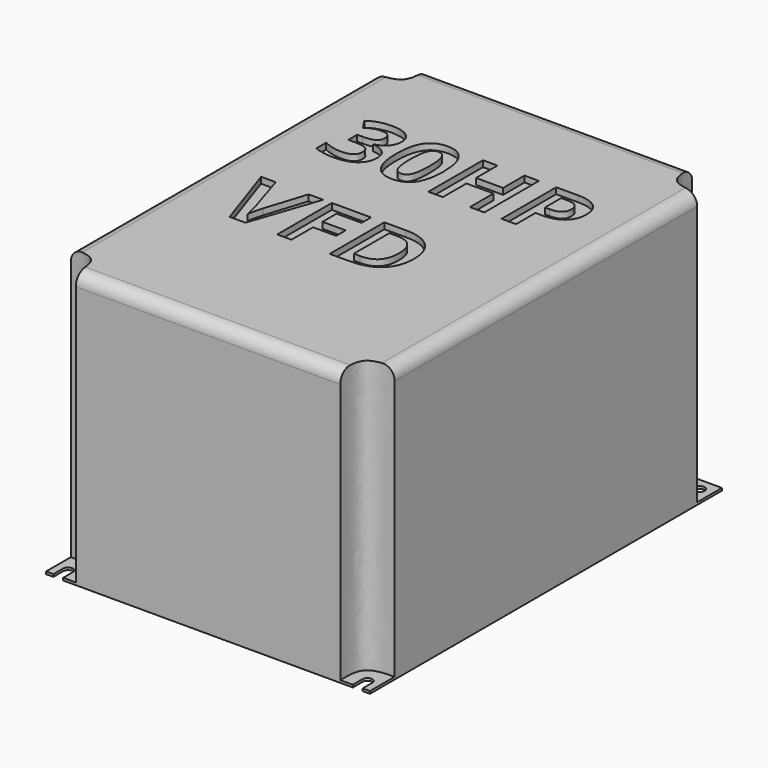
from build123d import *

# Parameters (mm, degrees)
F0_R         = 4
F1_DEPTH     = 2
F2_DEPTH     = 225
F3_R         = 10
F4_TEXT_SIZE = 78.2922502905
F5_DEPTH     = 5


# Not quite as in the source:
# - Text() gives the source's letters only with a copy of the font that has no kerning and outlines rounded to 1/6400 em; it was checked with that copy


with BuildPart() as f1:
    # F0 (on Top) → F1 (new body)
    with BuildSketch(Plane.XY):
        with BuildLine():
            Line((-108.2113981247, 180), (-132.5, 180))
            Line((-132.5, 180), (-132.5, 154.7320783138))
            add(Edge.make_bspline(
                [(-108.2113981247, 180), (-108.2113981247, 171.2072445138), (-108.3167336436, 156.7946357948), (-122.3416605587, 154.7320783138), (-132.5, 154.7320783138)],
                knots=[0, 0, 0, 0, 0.4931140285, 1, 1, 1, 1], degree=3))
        make_face()
        with Locations((-122.5, 170)):
            Circle(F0_R, mode=Mode.SUBTRACT)
        with BuildLine():
            Line((108.2113981247, 180), (-108.2113981247, 180))
            add(Edge.make_bspline(
                [(-108.2113981247, 180), (-108.2113981247, 171.2072445138), (-108.3167336436, 156.7946357948), (-122.3416605587, 154.7320783138), (-132.5, 154.7320783138)],
                knots=[0, 0, 0, 0, 0.4931140285, 1, 1, 1, 1], degree=3))
            Line((-132.5, 154.7320783138), (-132.5, -154.7320783138))
            add(Edge.make_bspline(
                [(-108.2113981247, -180), (-108.2113981247, -171.2072445138), (-108.3167336436, -156.7946357948), (-122.3416605587, -154.7320783138), (-132.5, -154.7320783138)],
                knots=[0, 0, 0, 0, 0.4931140285, 1, 1, 1, 1], degree=3))
            Line((-108.2113981247, -180), (108.2113981247, -180))
            add(Edge.make_bspline(
                [(108.2113981247, -180), (108.2113981247, -171.2072445138), (108.3167336436, -156.7946357948), (122.3416605587, -154.7320783138), (132.5, -154.7320783138)],
                knots=[0, 0, 0, 0, 0.4931140285, 1, 1, 1, 1], degree=3))
            Line((132.5, -154.7320783138), (132.5, 154.7320783138))
            add(Edge.make_bspline(
                [(108.2113981247, 180), (108.2113981247, 171.2072445138), (108.3167336436, 156.7946357948), (122.3416605587, 154.7320783138), (132.5, 154.7320783138)],
                knots=[0, 0, 0, 0, 0.4931140285, 1, 1, 1, 1], degree=3))
        make_face()
        with BuildLine():
            Line((132.5, 180), (108.2113981247, 180))
            add(Edge.make_bspline(
                [(108.2113981247, 180), (108.2113981247, 171.2072445138), (108.3167336436, 156.7946357948), (122.3416605587, 154.7320783138), (132.5, 154.7320783138)],
                knots=[0, 0, 0, 0, 0.4931140285, 1, 1, 1, 1], degree=3))
            Line((132.5, 154.7320783138), (132.5, 180))
        make_face()
        with Locations((122.5, 170)):
            Circle(F0_R, mode=Mode.SUBTRACT)
        with BuildLine():
            Line((132.5, -180), (132.5, -154.7320783138))
            add(Edge.make_bspline(
                [(108.2113981247, -180), (108.2113981247, -171.2072445138), (108.3167336436, -156.7946357948), (122.3416605587, -154.7320783138), (132.5, -154.7320783138)],
                knots=[0, 0, 0, 0, 0.4931140285, 1, 1, 1, 1], degree=3))
            Line((108.2113981247, -180), (118.5, -180))
            Line((118.5, -180), (118.5, -170))
            ThreePointArc((118.5, -170), (122.5, -166), (126.5, -170))
            Line((126.5, -170), (126.5, -180))
            Line((126.5, -180), (132.5, -180))
        make_face()
        with BuildLine():
            add(Edge.make_bspline(
                [(-108.2113981247, -180), (-108.2113981247, -171.2072445138), (-108.3167336436, -156.7946357948), (-122.3416605587, -154.7320783138), (-132.5, -154.7320783138)],
                knots=[0, 0, 0, 0, 0.4931140285, 1, 1, 1, 1], degree=3))
            Line((-132.5, -154.7320783138), (-132.5, -180))
            Line((-132.5, -180), (-126.5, -180))
            Line((-126.5, -180), (-126.5, -170))
            ThreePointArc((-126.5, -170), (-122.5, -166), (-118.5, -170))
            Line((-118.5, -170), (-118.5, -180))
            Line((-118.5, -180), (-108.2113981247, -180))
        make_face()
    extrude(amount=F1_DEPTH)

    # F0 (on Top) → F2 (join)
    with BuildSketch(Plane.XY):
        with BuildLine():
            Line((108.2113981247, 180), (-108.2113981247, 180))
            add(Edge.make_bspline(
                [(-108.2113981247, 180), (-108.2113981247, 171.2072445138), (-108.3167336436, 156.7946357948), (-122.3416605587, 154.7320783138), (-132.5, 154.7320783138)],
                knots=[0, 0, 0, 0, 0.4931140285, 1, 1, 1, 1], degree=3))
            Line((-132.5, 154.7320783138), (-132.5, -154.7320783138))
            add(Edge.make_bspline(
                [(-108.2113981247, -180), (-108.2113981247, -171.2072445138), (-108.3167336436, -156.7946357948), (-122.3416605587, -154.7320783138), (-132.5, -154.7320783138)],
                knots=[0, 0, 0, 0, 0.4931140285, 1, 1, 1, 1], degree=3))
            Line((-108.2113981247, -180), (108.2113981247, -180))
            add(Edge.make_bspline(
                [(108.2113981247, -180), (108.2113981247, -171.2072445138), (108.3167336436, -156.7946357948), (122.3416605587, -154.7320783138), (132.5, -154.7320783138)],
                knots=[0, 0, 0, 0, 0.4931140285, 1, 1, 1, 1], degree=3))
            Line((132.5, -154.7320783138), (132.5, 154.7320783138))
            add(Edge.make_bspline(
                [(108.2113981247, 180), (108.2113981247, 171.2072445138), (108.3167336436, 156.7946357948), (122.3416605587, 154.7320783138), (132.5, 154.7320783138)],
                knots=[0, 0, 0, 0, 0.4931140285, 1, 1, 1, 1], degree=3))
        make_face()
    extrude(amount=F2_DEPTH)

    # F3
    f3_edges = [f1.edges().sort_by_distance(p)[0] for p in [
        (0, 180, 225),
        (-132.5, 0, 225),
        (132.5, 0, 225),
        (0, -180, 225),
    ]]
    fillet(f3_edges, radius=F3_R)

    # F4 (on face) → F5 (cut)
    with BuildSketch(Plane.XY.offset(225)):
        with Locations((-98.7734862093, 48.3030493487)):
            Text('30HP', F4_TEXT_SIZE, font='Open Sans', font_style=FontStyle.BOLD, text_align=(TextAlign.LEFT, TextAlign.BOTTOM))
        with Locations((-98.7734862093, -58.1744110464)):
            Text('VFD', F4_TEXT_SIZE, font='Open Sans', font_style=FontStyle.BOLD, text_align=(TextAlign.LEFT, TextAlign.BOTTOM))
    extrude(amount=-F5_DEPTH, mode=Mode.SUBTRACT)


solid = f1.part
